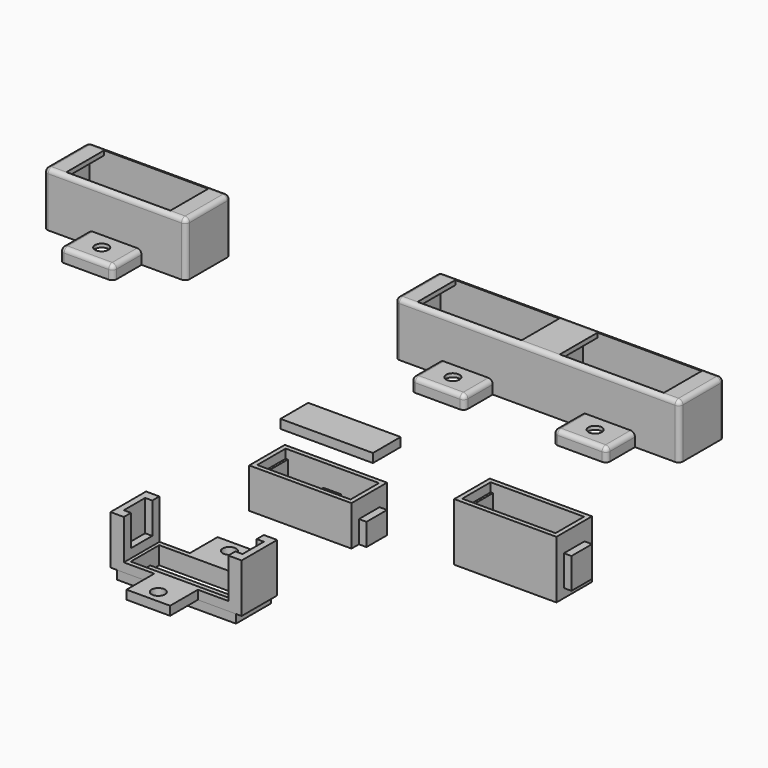
from build123d import *

# Parameters (mm, degrees)
F0_W      = 22
F0_H      = 2.5
F0_W_2    = 1
F0_H_2    = 10
F0_W_3    = 9.8
F0_H_3    = 7.8
F0_R      = 1.5
F2_DEPTH  = 1
F4_DEPTH  = 12.2
F5_T      = -1
F6_W      = 12
F6_H      = 8
F7_DEPTH  = 11.2
F9_W      = 1
F9_H      = 11.2
F10_DEPTH = 16
F11_W     = 30
F11_H     = 10.6
F12_DEPTH = 25
F13_W     = 10
F13_H     = 7
F13_R     = 1.5
F13_W_2   = 12
F13_H_2   = 8
F14_DEPTH = 2
F15_W     = 10
F15_H     = 26.6
F16_DEPTH = 2.2
F17_W     = 10.6
F17_H     = 1
F19_DEPTH = 3.3
F18_W     = 10.6
F18_H     = 1
F20_DEPTH = 3.3
F21_W     = 26.8
F21_H     = 9.8
F21_W_2   = 22
F21_H_2   = 2.5
F22_DEPTH = 2
F23_W     = 22
F23_H     = 8
F24_DEPTH = 2
F3_W      = 3
F3_H      = 10
F25_DEPTH = 10
F26_W     = 25.1
F26_H     = 6
F26_W_2   = 1.6
F27_DEPTH = 7
F28_W     = 8
F28_H     = 8
F28_W_2   = 1.7
F28_H_2   = 5.8
F29_DEPTH = 1
F31_DEPTH = 5
F32_DEPTH = 3
F33_DEPTH = 1
F34_W     = 23
F34_H     = 1
F35_DEPTH = 10
F36_R     = 1
F38_R     = 0.99999
F40_R     = 0.99999
F41_W     = 20.8
F41_H     = 7.8
F42_DEPTH = 2
F43_DEPTH = 3
F44_W     = 6.3
F44_H     = 6.3
F45_DEPTH = 1.5
F46_W     = 2
F46_H     = 2.5
F47_DEPTH = 3
F48_DEPTH = 1
F49_W     = 1.7
F49_H     = 5.8
F49_W_2   = 21
F49_H_2   = 8
F50_DEPTH = 9
F51_W     = 1.7
F51_H     = 5.8
F52_DEPTH = 2.1
F53_DEPTH = 2
F54_W     = 21
F54_H     = 8
F55_DEPTH = 2
F56_W     = 0.5
F56_H     = 8
F57_DEPTH = 13
F58_W     = 0.5
F58_H     = 8
F58_W_2   = 20
F59_DEPTH = 2


# Not quite as in the source:
# - a fillet or chamfer is up to 0.001 mm smaller than in the source, because OpenCascade refuses the exact size


with BuildPart() as f2:
    # F0 (on Top) → F2 (new body)
    with BuildSketch(Plane.XY):
        Polygon((-85.7184315681, -5), (-76.8684315681, -5), (-76.8684315681, 5), (-85.7184315681, 5), (-95.5184315681, 5), (-104.3684315681, 5), (-104.3684315681, -5), (-95.5184315681, -5), align=None)
        with Locations((-90.6184315681, -2.75)):
            Rectangle(F0_W, F0_H, mode=Mode.SUBTRACT)
        with Locations((-90.6184315681, 2.75)):
            Rectangle(F0_W, F0_H, mode=Mode.SUBTRACT)
        with Locations((-104.8684315681, 0)):
            Rectangle(F0_W_2, F0_H_2)
        with Locations((-76.3684315681, 0)):
            Rectangle(F0_W_2, F0_H_2)
        with Locations((-90.6184315681, 8.9)):
            Rectangle(F0_W_3, F0_H_3)
        with Locations((-90.6184315681, 10)):
            Circle(F0_R, mode=Mode.SUBTRACT)
        with Locations((-90.6184315681, -8.9)):
            Rectangle(F0_W_3, F0_H_3)
        with Locations((-90.6184315681, -10)):
            Circle(F0_R, mode=Mode.SUBTRACT)
    extrude(amount=F2_DEPTH)

    # F21 (on face) → F22 (join)
    with BuildSketch(Plane.XY):
        with Locations((-90.6184315681, 0)):
            Rectangle(F21_W, F21_H)
        with Locations((-90.6184315681, -2.75)):
            Rectangle(F21_W_2, F21_H_2, mode=Mode.SUBTRACT)
        with Locations((-90.6184315681, 2.75)):
            Rectangle(F21_W_2, F21_H_2, mode=Mode.SUBTRACT)
    extrude(amount=-F22_DEPTH)

    # F23 (on face) → F24 (cut)
    with BuildSketch(Plane.XY.offset(1)):
        with Locations((-90.6184315681, 0)):
            Rectangle(F23_W, F23_H)
    extrude(amount=-F24_DEPTH, mode=Mode.SUBTRACT)

    # F3 (on face) → F25 (join)
    with BuildSketch(Plane.XY.offset(1)):
        with Locations((-103.8684315681, 0)):
            Rectangle(F3_W, F3_H)
        with Locations((-77.3684315681, 0)):
            Rectangle(F3_W, F3_H)
    extrude(amount=F25_DEPTH)

    # F26 (on face) → F27 (cut)
    with BuildSketch(Plane.XY.offset(11)):
        with Locations((-89.8184315681, 0)):
            Rectangle(F26_W, F26_H)
        with Locations((-103.1684315681, 0)):
            Rectangle(F26_W_2, F26_H)
    extrude(amount=-F27_DEPTH, mode=Mode.SUBTRACT)

    # F33 (add): a face of the model
    f33_faces = [f2.faces().sort_by_distance(p)[0] for p in [
        (-98.9434315681, 4.6524931655, 1),
    ]]
    extrude(f33_faces, amount=F33_DEPTH)


with BuildPart() as f4:
    # F1 (on Top) → F4 (new body)
    with BuildSketch(Plane.XY):
        Polygon((-94.0465646753, 88.333089388), (-84.0465646753, 88.333089388), (-84.0465646753, 100.933089388), (-94.0465646753, 100.933089388), (-94.0465646753, 108.933089388), (-106.0465646753, 108.933089388), (-106.0465646753, 100.933089388), (-116.0465646753, 100.933089388), (-116.0465646753, 88.333089388), (-106.0465646753, 88.333089388), (-106.0465646753, 80.333089388), (-94.0465646753, 80.333089388), align=None)
    extrude(amount=F4_DEPTH)

    # F5
    f5_openings = [f4.faces().sort_by_distance(p)[0] for p in [
        (-100.046565, 94.633089, 0),
    ]]
    offset(amount=F5_T, openings=f5_openings, kind=Kind.INTERSECTION)

    # F6 (on face) → F7 (cut)
    with BuildSketch(Plane.XY.offset(12.2)):
        Polygon((-106.0465646753, 88.333089388), (-110.0465646753, 88.333089388), (-110.0465646753, 79.5402535319), (-90.0465646753, 79.5402535319), (-90.0465646753, 88.333089388), (-94.0465646753, 88.333089388), (-94.0465646753, 80.333089388), (-106.0465646753, 80.333089388), align=None)
        Polygon((-85.3086039424, 109.6437925995), (-110.0465646753, 109.6437925995), (-110.0465646753, 100.933089388), (-106.0465646753, 100.933089388), (-106.0465646753, 108.933089388), (-94.0465646753, 108.933089388), (-94.0465646753, 100.933089388), (-85.3086039424, 100.933089388), align=None)
        with Locations((-100.0465646753, 104.933089388)):
            Rectangle(F6_W, F6_H)
        with Locations((-100.0465646753, 84.333089388)):
            Rectangle(F6_W, F6_H)
    extrude(amount=-F7_DEPTH, mode=Mode.SUBTRACT)

    # F9 (on face) + F8 (on face) → F10 (join)
    with BuildSketch(Plane(origin=(-95.0465646753, 0, 0), x_dir=(0, -1, 0), z_dir=(-1, 0, 0))):
        with Locations((-100.433089388, 5.6)):
            Rectangle(F9_W, F9_H)
    with BuildSketch(Plane(origin=(-95.0465646753, 0, 0), x_dir=(0, -1, 0), z_dir=(-1, 0, 0))):
        Polygon((-88.333089388, 1), (-88.333089388, 11.2), (-89.333089388, 11.2), (-89.333089388, 0), (-88.333089388, 0), align=None)
    extrude(amount=F10_DEPTH)

    # F11 (on face) → F12 (cut)
    with BuildSketch(Plane.XY.offset(12.2)):
        with Locations((-100.0465646753, 94.633089388)):
            Rectangle(F11_W, F11_H)
    extrude(amount=-F12_DEPTH, mode=Mode.SUBTRACT)

    # F13 (on face) → F14 (join)
    with BuildSketch(Plane.XY.offset(1)):
        with Locations((-100.0465646753, 104.433089388)):
            Rectangle(F13_W, F13_H)
        with Locations((-100.0465646753, 104.633089388)):
            Circle(F13_R, mode=Mode.SUBTRACT)
        Polygon((-94.0465646753, 108.933089388), (-106.0465646753, 108.933089388), (-106.0465646753, 100.933089388), (-105.0465646753, 100.933089388), (-105.0465646753, 107.933089388), (-95.0465646753, 107.933089388), (-95.0465646753, 100.933089388), (-94.0465646753, 100.933089388), align=None)
        with Locations((-100.0465646753, 84.333089388)):
            Rectangle(F13_W_2, F13_H_2)
        with Locations((-100.0465646753, 84.633089388)):
            Circle(F13_R, mode=Mode.SUBTRACT)
    extrude(amount=F14_DEPTH)

    # F15 (on face) → F16 (cut)
    with BuildSketch(Plane.XY):
        with Locations((-100.0465646753, 94.633089388)):
            Rectangle(F15_W, F15_H)
    extrude(amount=F16_DEPTH, mode=Mode.SUBTRACT)

    # F17 (on face) → F19 (join)
    with BuildSketch(Plane.YZ.offset(-115.0465646753)):
        with Locations((94.633089388, 11.7)):
            Rectangle(F17_W, F17_H)
    extrude(amount=F19_DEPTH)

    # F18 (on face) → F20 (join)
    with BuildSketch(Plane(origin=(-85.0465646753, 0, 0), x_dir=(0, -1, 0), z_dir=(-1, 0, 0))):
        with Locations((-94.633089388, 11.7)):
            Rectangle(F18_W, F18_H)
    extrude(amount=F20_DEPTH)

    # F36
    f36_edges = [f4.edges().sort_by_distance(p)[0] for p in [
        (-106.046565, 84.333089, 3),
        (-94.046565, 84.333089, 3),
        (-100.046565, 80.333089, 3),
        (-106.046565, 80.333089, 1.5),
        (-94.046565, 80.333089, 1.5),
        (-94.046565, 104.933089, 3),
        (-94.046565, 108.933089, 1.5),
        (-100.046565, 108.933089, 3),
        (-106.046565, 104.933089, 3),
        (-106.046565, 108.933089, 1.5),
    ]]
    fillet(f36_edges, radius=F36_R)


with BuildPart() as f29:
    # F28 (on Top) → F29 (new body)
    with BuildSketch(Plane.XY):
        Polygon((-103.418990016, 30.5717597306), (-80.418990016, 30.5717597306), (-80.418990016, 33.6717597306), (-80.418990016, 39.4717597306), (-80.418990016, 42.5717597306), (-103.418990016, 42.5717597306), (-103.418990016, 39.4717597306), (-103.418990016, 33.6717597306), align=None)
        with Locations((-97.918990016, 36.5717597306)):
            Rectangle(F28_W, F28_H, mode=Mode.SUBTRACT)
        with Locations((-85.918990016, 36.5717597306)):
            Rectangle(F28_W, F28_H, mode=Mode.SUBTRACT)
        with Locations((-104.268990016, 36.5717597306)):
            Rectangle(F28_W_2, F28_H_2)
        with Locations((-79.568990016, 36.5717597306)):
            Rectangle(F28_W_2, F28_H_2)
    extrude(amount=F29_DEPTH)

    # F30 (on face) → F31 (join)
    with BuildSketch(Plane.XY.offset(1)):
        Polygon((-80.418990016, 41.5717597306), (-103.418990016, 41.5717597306), (-103.418990016, 39.4717597306), (-103.418990016, 33.6717597306), (-103.418990016, 31.5717597306), (-80.418990016, 31.5717597306), (-80.418990016, 33.6717597306), (-80.418990016, 39.4717597306), align=None)
        Polygon((-102.418990016, 32.5717597306), (-102.418990016, 40.5717597306), (-101.918990016, 40.5717597306), (-93.918990016, 40.5717597306), (-89.918990016, 40.5717597306), (-81.918990016, 40.5717597306), (-81.418990016, 40.5717597306), (-81.418990016, 32.5717597306), (-81.918990016, 32.5717597306), (-89.918990016, 32.5717597306), (-93.918990016, 32.5717597306), (-101.918990016, 32.5717597306), align=None, mode=Mode.SUBTRACT)
    extrude(amount=F31_DEPTH)

    # F32 (add): faces of the model
    f32_faces = [f29.faces().sort_by_distance(p)[0] for p in [
        (-81.668990016, 36.5717597306, 1),
        (-102.168990016, 36.5717597306, 1),
    ]]
    extrude(f32_faces, amount=F32_DEPTH)

    # F34 (on face) → F35 (cut)
    with BuildSketch(Plane.XY.offset(6)):
        with Locations((-91.918990016, 42.0717597306)):
            Rectangle(F34_W, F34_H)
        with Locations((-91.918990016, 31.0717597306)):
            Rectangle(F34_W, F34_H)
    extrude(amount=-F35_DEPTH, mode=Mode.SUBTRACT)

    # F43 (add): a face of the model
    f43_faces = [f29.faces().sort_by_distance(p)[0] for p in [
        (-91.918990016, 36.5717597306, 0),
    ]]
    extrude(f43_faces, amount=F43_DEPTH)

    # F44 (on face) → F45 (cut)
    with BuildSketch(Plane(origin=(0, 0, -3), x_dir=(1, 0, 0), z_dir=(0, 0, -1))):
        with Locations((-91.918990016, -36.5717597306)):
            Rectangle(F44_W, F44_H)
    extrude(amount=-F45_DEPTH, mode=Mode.SUBTRACT)

    # F46 (on face) → F47 (cut)
    with BuildSketch(Plane(origin=(0, 0, -3), x_dir=(1, 0, 0), z_dir=(0, 0, -1))):
        with Locations((-91.918990016, -36.5717597306)):
            Rectangle(F46_W, F46_H)
    extrude(amount=-F47_DEPTH, mode=Mode.SUBTRACT)

    # F48 (add): faces of the model
    f48_faces = [f29.faces().sort_by_distance(p)[0] for p in [
        (-104.268990016, 36.5717597306, 1),
        (-79.568990016, 36.5717597306, 1),
    ]]
    extrude(f48_faces, amount=F48_DEPTH)


with BuildPart() as f37_1:
    # F37: copy of F4
    add(f4.part.moved(Location((-79, 0, 0))))

    # F38 (radius 1 in the source; OpenCascade refuses exactly that, so slightly less here)
    f38_edges = [f37_1.edges().sort_by_distance(p)[0] for p in [
        (-195.046565, 88.333089, 6.1),
        (-195.046565, 100.933089, 6.1),
        (-163.046565, 88.333089, 6.1),
        (-163.046565, 100.933089, 6.1),
        (-195.046565, 94.633089, 12.2),
        (-179.046565, 88.333089, 12.2),
        (-179.046565, 100.933089, 12.2),
        (-163.046565, 94.633089, 12.2),
    ]]
    fillet(f38_edges, radius=F38_R)


with BuildPart() as f4_1:
    add(f4.part)

    # F39: F4 across face
    add(f4.part.mirror(Plane(origin=(-84.0465646753, 94.633089388, 6.1), x_dir=(0, 1, 0), z_dir=(1, 0, 0))))

    # F40 (radius 1 in the source; OpenCascade refuses exactly that, so slightly less here)
    f40_edges = [f4_1.edges().sort_by_distance(p)[0] for p in [
        (-116.046565, 88.333089, 6.1),
        (-116.046565, 100.933089, 6.1),
        (-52.046565, 88.333089, 6.1),
        (-52.046565, 100.933089, 6.1),
        (-52.046565, 94.633089, 12.2),
        (-84.046565, 88.333089, 12.2),
        (-84.046565, 100.933089, 12.2),
        (-116.046565, 94.633089, 12.2),
    ]]
    fillet(f40_edges, radius=F40_R)


with BuildPart() as f42:
    # F41 (on Top) → F42 (new body)
    with BuildSketch(Plane.XY):
        with Locations((-104.6008812547, 58.7332594335)):
            Rectangle(F41_W, F41_H)
    extrude(amount=F42_DEPTH)


with BuildPart() as f50:
    # F49 (on Top) → F50 (new body)
    with BuildSketch(Plane.XY):
        with Locations((-62.1514464974, 41.5642715096)):
            Rectangle(F49_W, F49_H)
        Polygon((-61.3014464974, 36.5642715096), (-38.3014464974, 36.5642715096), (-38.3014464974, 38.6642715096), (-38.3014464974, 44.4642715096), (-38.3014464974, 46.5642715096), (-61.3014464974, 46.5642715096), (-61.3014464974, 44.4642715096), (-61.3014464974, 38.6642715096), align=None)
        with Locations((-49.8014464974, 41.5642715096)):
            Rectangle(F49_W_2, F49_H_2, mode=Mode.SUBTRACT)
        with Locations((-37.4514464974, 41.5642715096)):
            Rectangle(F49_W, F49_H)
    extrude(amount=F50_DEPTH)

    # F51 (on face) → F52 (cut)
    with BuildSketch(Plane.XY.offset(9)):
        with Locations((-62.1514464974, 41.5642715096)):
            Rectangle(F51_W, F51_H)
        with Locations((-37.4514464974, 41.5642715096)):
            Rectangle(F51_W, F51_H)
    extrude(amount=-F52_DEPTH, mode=Mode.SUBTRACT)

    # F53 (add): a face of the model
    f53_faces = [f50.faces().sort_by_distance(p)[0] for p in [
        (-49.8014464974, 46.3134727856, 9),
    ]]
    extrude(f53_faces, amount=F53_DEPTH)

    # F54 (on face) → F55 (join)
    with BuildSketch(Plane(origin=(0, 0, 0), x_dir=(1, 0, 0), z_dir=(0, 0, -1))):
        Polygon((-38.3014464974, -36.5642715096), (-61.3014464974, -36.5642715096), (-61.3014464974, -38.6642715096), (-61.3014464974, -44.4642715096), (-61.3014464974, -46.5642715096), (-38.3014464974, -46.5642715096), (-38.3014464974, -44.4642715096), (-38.3014464974, -38.6642715096), align=None)
        with Locations((-49.8014464974, -41.5642715096)):
            Rectangle(F54_W, F54_H, mode=Mode.SUBTRACT)
    extrude(amount=F55_DEPTH)

    # F56 (on face) → F57 (join)
    with BuildSketch(Plane.XY.offset(11)):
        with Locations((-60.0514464974, 41.5642715096)):
            Rectangle(F56_W, F56_H)
        with Locations((-39.5514464974, 41.5642715096)):
            Rectangle(F56_W, F56_H)
    extrude(amount=-F57_DEPTH)

    # F58 (on face) → F59 (cut)
    with BuildSketch(Plane.XY.offset(11)):
        with Locations((-60.0514464974, 41.5642715096)):
            Rectangle(F58_W, F58_H)
        with Locations((-49.8014464974, 41.5642715096)):
            Rectangle(F58_W_2, F58_H)
        with Locations((-39.5514464974, 41.5642715096)):
            Rectangle(F58_W, F58_H)
    extrude(amount=-F59_DEPTH, mode=Mode.SUBTRACT)


solid = Compound([f2.part, f29.part, f37_1.part, f4_1.part, f42.part, f50.part])
